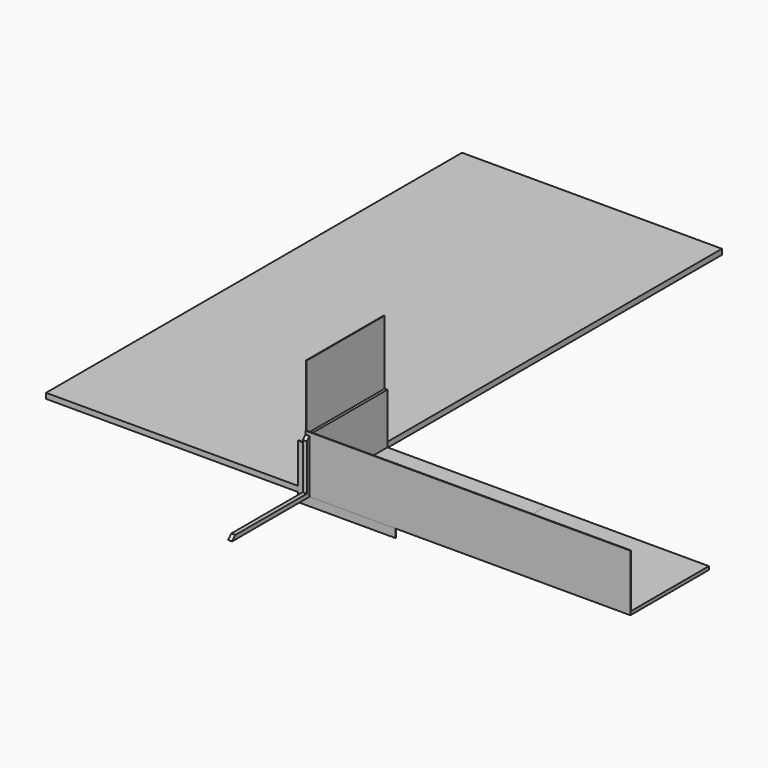
from build123d import *

# Parameters (mm, degrees)
F0_W      = 1524
F0_H      = 457.2
F1_DEPTH  = 15.875
F2_W      = 457.2
F2_H      = 254
F3_DEPTH  = 15.875
F4_W      = 101.6
F4_H      = 101.6
F5_DEPTH  = 76.2
F7_DEPTH  = 1524
F8_W      = 19.05
F8_H      = 19.05
F9_DEPTH  = 457.2
F10_SIZE  = 19.04999
F11_W     = 19.05
F11_H     = 19.05
F12_DEPTH = 254
F13_SIZE  = 19.04999
F14_W     = 457.2
F14_H     = 254
F15_DEPTH = 3.175
F16_W     = 457.2
F16_H     = 555.625
F17_DEPTH = 3.175
F18_W     = 1524
F18_H     = 266.7
F19_DEPTH = 3.175
F21_W     = 762
F21_H     = 457.2
F22_DEPTH = 15.875
F20_W     = 1219.2
F20_H     = 2438.4
F23_DEPTH = 25.4


# Not quite as in the source:
# - a fillet or chamfer is up to 0.001 mm smaller than in the source, because OpenCascade refuses the exact size


with BuildPart() as f1:
    # F0 (on Top) → F1 (new body)
    with BuildSketch(Plane.XY):
        with Locations((762, 228.6)):
            Rectangle(F0_W, F0_H)
    extrude(amount=F1_DEPTH)


with BuildPart() as f3:
    # F2 (on Right) → F3 (new body)
    with BuildSketch(Plane.YZ):
        with Locations((228.6, 127)):
            Rectangle(F2_W, F2_H)
    extrude(amount=F3_DEPTH)


with BuildPart() as f5:
    # F4 (on Top) → F5 (new body)
    with BuildSketch(Plane.XY):
        with Locations((50.8, 50.8)):
            Rectangle(F4_W, F4_H)
    extrude(amount=F5_DEPTH)


with BuildPart() as f7:
    # F6 (on Right) → F7 (new body)
    with BuildSketch(Plane.YZ):
        Polygon((0, 19.05), (0, 0), (19.05, 0), (19.05, 3.175), (3.175, 3.175), (3.175, 19.05), align=None)
    extrude(amount=F7_DEPTH)


with BuildPart() as f9:
    # F8 (on Front) → F9 (new body)
    with BuildSketch(Plane.XZ):
        with Locations((9.525, 9.525)):
            Rectangle(F8_W, F8_H)
    extrude(amount=F9_DEPTH)

    # F10 (size 19.05 in the source; OpenCascade refuses exactly that, so slightly less here)
    f10_edges = [f9.edges().sort_by_distance(p)[0] for p in [
        (9.525, -457.2, 19.05),
        (9.525, 0, 19.05),
    ]]
    chamfer(f10_edges, length=F10_SIZE)


with BuildPart() as f12:
    # F11 (on Top) → F12 (new body)
    with BuildSketch(Plane.XY):
        with Locations((9.525, -9.525)):
            Rectangle(F11_W, F11_H)
    extrude(amount=F12_DEPTH)

    # F13 (size 19.05 in the source; OpenCascade refuses exactly that, so slightly less here)
    f13_edges = [f12.edges().sort_by_distance(p)[0] for p in [
        (9.525, -19.05, 254),
        (9.525, -19.05, 0),
    ]]
    chamfer(f13_edges, length=F13_SIZE)


with BuildPart() as f15:
    # F14 (on Front) → F15 (new body)
    with BuildSketch(Plane.XZ):
        with Locations((194.4030308783, 87.2860808372)):
            Rectangle(F14_W, F14_H)
    extrude(amount=F15_DEPTH)


with BuildPart() as f17:
    # F16 (on Right) → F17 (new body)
    with BuildSketch(Plane.YZ):
        with Locations((228.6, 277.8125)):
            Rectangle(F16_W, F16_H)
    extrude(amount=F17_DEPTH)


with BuildPart() as f19:
    # F18 (on Front) → F19 (new body)
    with BuildSketch(Plane.XZ):
        with Locations((762, 133.35)):
            Rectangle(F18_W, F18_H)
    extrude(amount=F19_DEPTH)


with BuildPart() as f22:
    # F21 (on Top) → F22 (new body)
    with BuildSketch(Plane.XY):
        with Locations((381, 228.6)):
            Rectangle(F21_W, F21_H)
    extrude(amount=F22_DEPTH)


with BuildPart() as f23:
    # F20 (on Top) → F23 (new body)
    with BuildSketch(Plane.XY):
        with Locations((-609.6, 1219.2)):
            Rectangle(F20_W, F20_H)
    extrude(amount=F23_DEPTH)


solid = Compound([f1.part, f3.part, f5.part, f7.part, f9.part, f12.part, f15.part, f17.part, f19.part, f22.part, f23.part])
